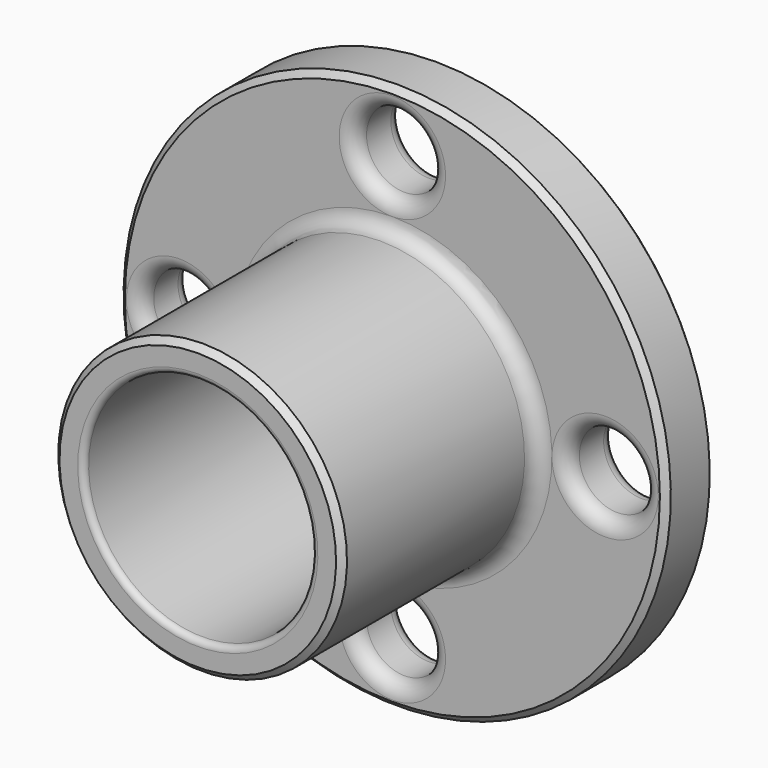
from build123d import *

# Parameters (mm, degrees)
F2_R     = 12.5
F3_DEPTH = 20
F4_SIZE  = 2
F5_R     = 4.99999
F6_R     = 10
F7_R     = 2


# Not quite as in the source:
# - a fillet or chamfer is up to 0.001 mm smaller than in the source, because OpenCascade refuses the exact size


with BuildPart() as f1:
    # F0 (on Right) → F1 (revolve)
    with BuildSketch(Plane.YZ):
        Polygon((-20, 47.5), (-100, 47.5), (-100, 37.5), (0, 37.5), (0, 90), (-20, 90), align=None)
    revolve(axis=Axis((0, -59.8429322233, 0), (0, -1, 0)))

    # F2 (on face) → F3 (cut, through all)
    with BuildSketch(Plane.XZ.offset(20)):
        with Locations((0, 70)):
            Circle(F2_R)
        with Locations((-70, 0)):
            Circle(F2_R)
        with Locations((0, -70)):
            Circle(F2_R)
        with Locations((70, 0)):
            Circle(F2_R)
    extrude(amount=-F3_DEPTH, mode=Mode.SUBTRACT)

    # F4
    f4_edges = [f1.edges().sort_by_distance(p)[0] for p in [
        (0, -100, -47.5),
        (0, -20, -90),
        (0, 0, -90),
    ]]
    chamfer(f4_edges, length=F4_SIZE)

    # F5 (radius 5 in the source; OpenCascade refuses exactly that, so slightly less here)
    f5_edges = [f1.edges().sort_by_distance(p)[0] for p in [
        (0, -20, -47.5),
        (-12.5, -20, 70),
        (57.5, -20, 0),
        (-12.5, -20, -70),
        (-82.5, -20, 0),
        (-82.5, 0, 0),
        (-12.5, 0, 70),
        (57.5, 0, 0),
        (-12.5, 0, -70),
    ]]
    fillet(f5_edges, radius=F5_R)

    # F6
    f6_edges = [f1.edges().sort_by_distance(p)[0] for p in [
        (0, 0, -37.5),
    ]]
    fillet(f6_edges, radius=F6_R)

    # F7
    f7_edges = [f1.edges().sort_by_distance(p)[0] for p in [
        (0, -100, -37.5),
    ]]
    fillet(f7_edges, radius=F7_R)


solid = f1.part
